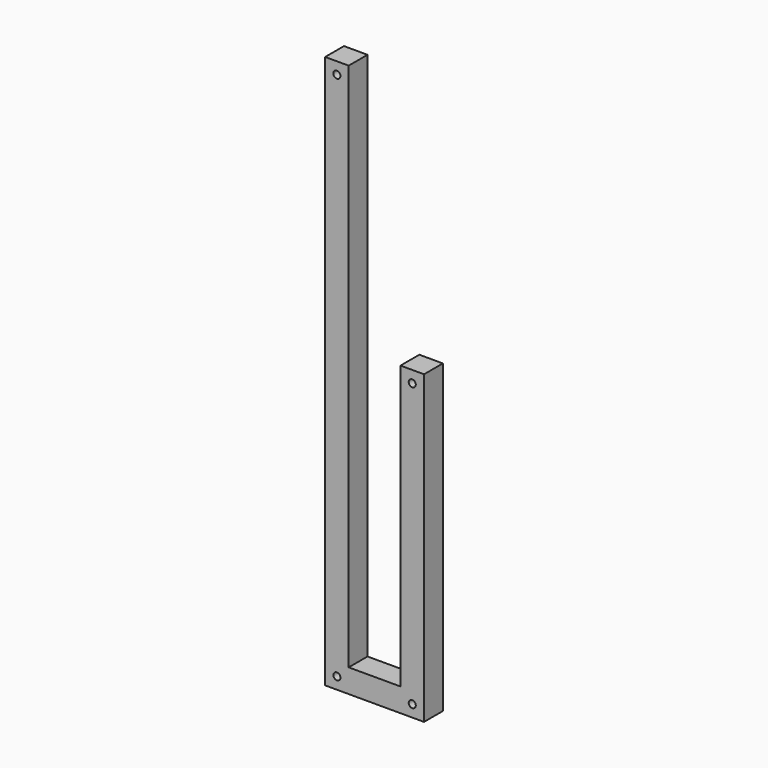
from build123d import *

# Parameters (mm, degrees)
F0_R     = 1.5
F0_W     = 22
F0_H     = 10
F1_DEPTH = 5
F2_DEPTH = 5


# Not quite as in the source:
# - a feature names something its author has since deleted; it is built from what else it names


with BuildPart() as f1:
    # F0 (on Front) → F1 (new body, symmetric)
    with BuildSketch(Plane.XZ):
        Polygon((10, 147.8899265081), (0, 147.8899265081), (0, -87.1100734919), (10, -87.1100734919), (10, -77.1100734919), align=None)
        with Locations((5, -82.1100734919)):
            Circle(F0_R, mode=Mode.SUBTRACT)
        with Locations((5, 142.8899265081)):
            Circle(F0_R, mode=Mode.SUBTRACT)
        with Locations((21, -82.1100734919)):
            Rectangle(F0_W, F0_H)
        Polygon((32, 42.8899265081), (32, -77.1100734919), (32, -87.1100734919), (42, -87.1100734919), (42, 42.8899265081), align=None)
        with Locations((37, -82.1100734919)):
            Circle(F0_R, mode=Mode.SUBTRACT)
        with Locations((37, 37.8899265081)):
            Circle(F0_R, mode=Mode.SUBTRACT)
    extrude(amount=F1_DEPTH, both=True)

    # F0 (on Front) → F2 (cut, symmetric)
    with BuildSketch(Plane.XZ):
        with Locations((5, -82.1100734919)):
            Circle(F0_R)
        with Locations((37, -82.1100734919)):
            Circle(F0_R)
        with Locations((37, 37.8899265081)):
            Circle(F0_R)
        with Locations((5, 142.8899265081)):
            Circle(F0_R)
    extrude(amount=F2_DEPTH, both=True, mode=Mode.SUBTRACT)


solid = f1.part
